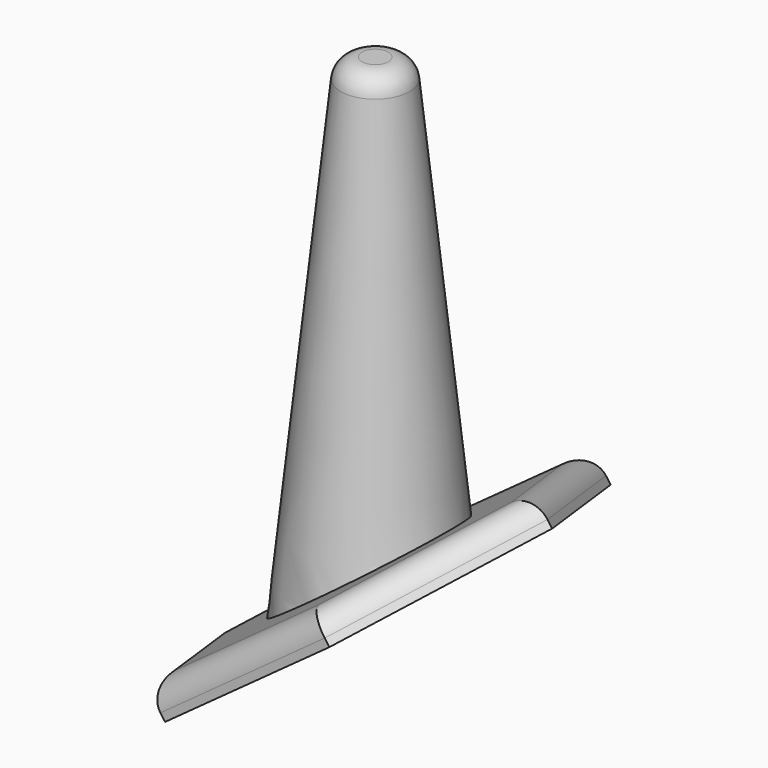
from build123d import *

# Parameters (mm, degrees)
F3_DEPTH      = 11.001
F3_DEPTH_BACK = 11.001
F5_DEPTH      = 4
F6_R          = 3
F7_R          = 2.69


with BuildPart() as f1:
    # F0 (on Front) → F1 (revolve)
    with BuildSketch(Plane.XZ):
        Polygon((-4.066010414, 66), (-11, 0), (0, 0), (0, 66), align=None)
    revolve(axis=Axis((0, 0, 33), (0, 0, -1)))

    # F2 (on Front) → F3 (cut, two sides)
    with BuildSketch(Plane.XZ) as f3_sk:
        Polygon((40.7802015543, 39.7115387022), (-13.9303933829, 0), (40.7802015543, 0), align=None)
    extrude(amount=-F3_DEPTH, mode=Mode.SUBTRACT)
    extrude(f3_sk.sketch, amount=F3_DEPTH_BACK, mode=Mode.SUBTRACT)

    # F4 (on face) → F5 (join)
    with BuildSketch(Plane(origin=(-4.8068030747, 0, 6.6223335725), x_dir=(0.8092844528, 0, 0.5874169511), z_dir=(0.5874169511, 0, -0.8092844528))):
        Polygon((-7.7040281941, -22), (17.6993836503, -22), (30.4010895725, 0), (17.6993836503, 22), (-7.7040281941, 22), (-20.4057341162, 0), align=None)
    extrude(amount=F5_DEPTH)

    # F6
    f6_edges = [f1.edges().sort_by_distance(p)[0] for p in [
        (-0.76226, 22, 9.558054),
        (14.65668, 11, 20.74985),
        (14.65668, -11, 20.74985),
        (-0.76226, -22, 9.558054),
        (-16.1812, -11, -1.633742),
        (-16.1812, 11, -1.633742),
    ]]
    fillet(f6_edges, radius=F6_R)

    # F7
    f7_edges = [f1.edges().sort_by_distance(p)[0] for p in [
        (4.06601, 0, 66),
    ]]
    fillet(f7_edges, radius=F7_R)


solid = f1.part
